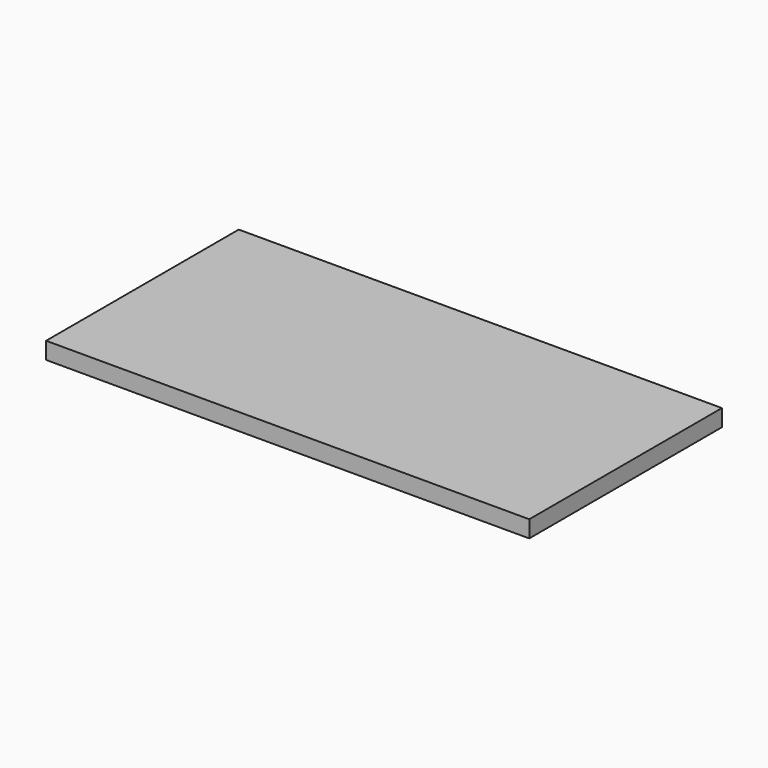
from build123d import *

# Parameters (mm, degrees)
F1_W         = 181.5760433674
F1_H         = 90.4911458492
F2_DEPTH     = 6.35
F0_W         = 130.5429952645
F0_H         = 9.9406372756
F0_TEXT_SIZE = 56.3406278031
F3_DEPTH     = 2.54


# Not quite as in the source:
# - Text() gives the source's letters only with a copy of the font that has no kerning and outlines rounded to 1/6400 em; it was checked with that copy


with BuildPart() as f2:
    # F1 (on Top) → F2 (new body)
    with BuildSketch(Plane.XY):
        Rectangle(F1_W, F1_H)
    extrude(amount=F2_DEPTH)

    # F0 (on Top) → F3 (join)
    with BuildSketch(Plane.XY):
        with Locations((-0.9185961235, 33.82241074)):
            Rectangle(F0_W, F0_H)
        with Locations((-0.9185961235, -32.1252280846)):
            Rectangle(F0_W, F0_H)
        with Locations((-66.1900937557, -19.421476271)):
            Text('KSTC', F0_TEXT_SIZE, font='Open Sans', text_align=(TextAlign.LEFT, TextAlign.BOTTOM))
    extrude(amount=-F3_DEPTH)


solid = f2.part
